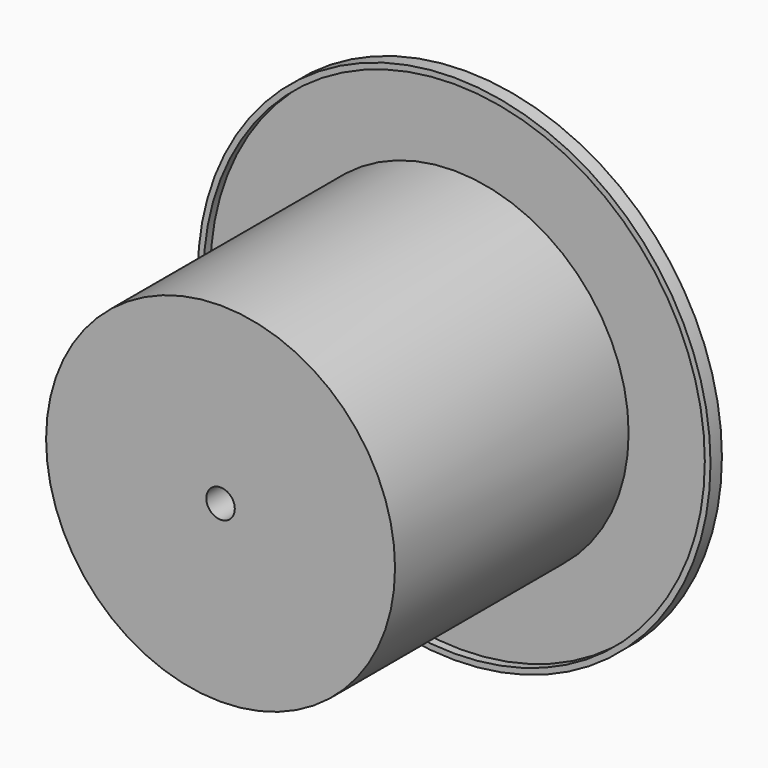
from build123d import *

# Parameters (mm, degrees)
F0_R     = 114.3
F0_R_2   = 77.7875
F1_DEPTH = 6.35
F2_DEPTH = 203.2
F3_DEPTH = 101.6
F4_R     = 6.35
F5_DEPTH = 101.601
F6_T     = -2.54
F7_DEPTH = 9.525
F8_DEPTH = 25.4


# Not quite as in the source:
# - a shell that OpenCascade refuses in one call is made with other operations: the cavity is built on its own and cut out


with BuildPart() as f1:
    # F0 (on Front) → F1 (new body)
    with BuildSketch(Plane.XZ):
        Circle(F0_R)
        Circle(F0_R_2, mode=Mode.SUBTRACT)
    extrude(amount=F1_DEPTH)

    # F0 (on Front) → F2 (join)
    with BuildSketch(Plane.XZ):
        Circle(F0_R_2)
    extrude(amount=F2_DEPTH)

    # F3 (cut): a face of the model
    f3_faces = [f1.faces().sort_by_distance(p)[0] for p in [
        (0, -203.2, 0),
    ]]
    extrude(f3_faces, amount=-F3_DEPTH, mode=Mode.SUBTRACT)

    # F4 (on face) → F5 (cut, through all)
    with BuildSketch(Plane.XZ.offset(101.6)):
        Circle(F4_R)
    extrude(amount=-F5_DEPTH, mode=Mode.SUBTRACT)

    # F6: a shell. OpenCascade refuses it in one call, so the cavity is built on its own and cut out:
    # the body offset inwards by the wall thickness, plus a prism from it out through each open face.
    f6_core = offset(f1.part, amount=F6_T, kind=Kind.INTERSECTION, mode=Mode.PRIVATE)
    f6_exits = [f6_core.faces().sort_by_distance(p)[0] for p in [
        (-78.40855, -3.81, 0),
    ]]
    add(f6_core, mode=Mode.SUBTRACT)
    extrude(f6_exits, amount=-F6_T, mode=Mode.SUBTRACT)

    # F7 (add): a face of the model
    f7_faces = [f1.faces().sort_by_distance(p)[0] for p in [
        (-75.5873372503, -101.6, 0),
    ]]
    extrude(f7_faces, amount=F7_DEPTH)

    # F8 (add): a face of the model
    f8_faces = [f1.faces().sort_by_distance(p)[0] for p in [
        (-75.5873372503, -111.125, 0),
    ]]
    extrude(f8_faces, amount=F8_DEPTH)


solid = f1.part
